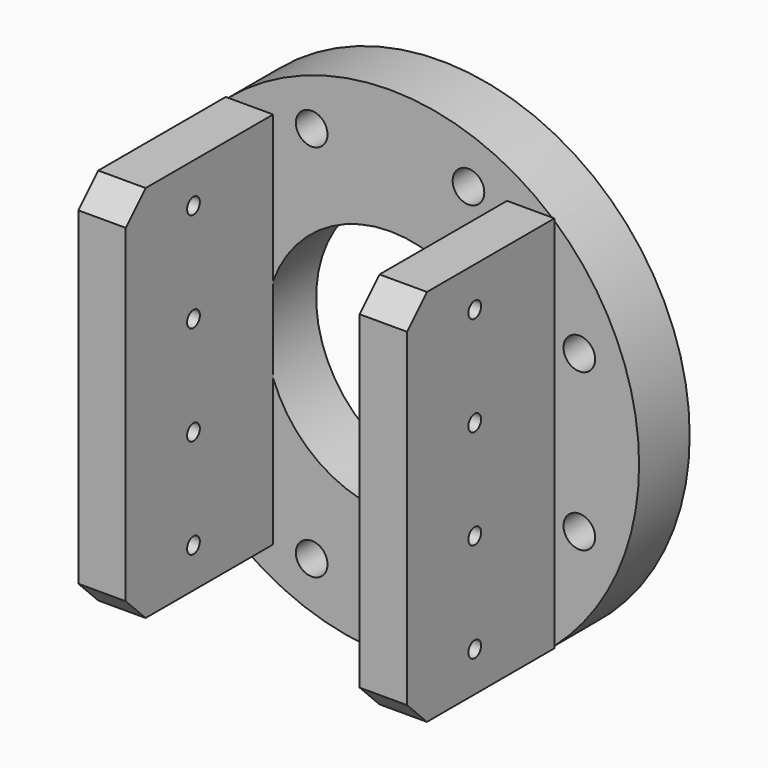
from build123d import *

# Parameters (mm, degrees)
F0_R     = 50
F0_R_2   = 3.175
F0_R_3   = 25
F1_DEPTH = 12.7
F2_W     = 9.525
F2_H     = 76
F3_DEPTH = 37
F4_R     = 1.6
F5_DEPTH = 83.001
F6_SIZE  = 5


# Not quite as in the source:
# - a feature names something its author has since deleted; it is built from what else it names


with BuildPart() as f1:
    # F0 (on Front) → F1 (new body)
    with BuildSketch(Plane.XZ):
        Circle(F0_R)
        with Locations((-15.7401153702, -38)):
            Circle(F0_R_2, mode=Mode.SUBTRACT)
        with Locations((-38, -15.7401153702)):
            Circle(F0_R_2, mode=Mode.SUBTRACT)
        with Locations((15.7401153702, -38)):
            Circle(F0_R_2, mode=Mode.SUBTRACT)
        with Locations((38, -15.7401153702)):
            Circle(F0_R_2, mode=Mode.SUBTRACT)
        with Locations((-38, 15.7401153702)):
            Circle(F0_R_2, mode=Mode.SUBTRACT)
        with Locations((-15.7401153702, 38)):
            Circle(F0_R_2, mode=Mode.SUBTRACT)
        Circle(F0_R_3, mode=Mode.SUBTRACT)
        with Locations((38, 15.7401153702)):
            Circle(F0_R_2, mode=Mode.SUBTRACT)
        with Locations((15.7401153702, 38)):
            Circle(F0_R_2, mode=Mode.SUBTRACT)
    extrude(amount=F1_DEPTH)

    # F2 (on face) → F3 (join)
    with BuildSketch(Plane.XZ.offset(12.7)):
        with Locations((-28.2375, 0)):
            Rectangle(F2_W, F2_H)
        with Locations((28.2375, 0)):
            Rectangle(F2_W, F2_H)
    extrude(amount=F3_DEPTH)

    # F4 (on face) → F5 (cut, through all)
    with BuildSketch(Plane(origin=(-33, 0, 0), x_dir=(0, -1, 0), z_dir=(-1, 0, 0))):
        with Locations((32.7, 30)):
            Circle(F4_R)
        with Locations((32.7, 10)):
            Circle(F4_R)
        with Locations((32.7, -10)):
            Circle(F4_R)
        with Locations((32.7, -30)):
            Circle(F4_R)
    extrude(amount=-F5_DEPTH, mode=Mode.SUBTRACT)

    # F6
    f6_edges = [f1.edges().sort_by_distance(p)[0] for p in [
        (-28.2375, -49.7, -38),
        (28.2375, -49.7, -38),
        (-28.2375, -49.7, 38),
        (28.2375, -49.7, 38),
    ]]
    chamfer(f6_edges, length=F6_SIZE)


solid = f1.part
